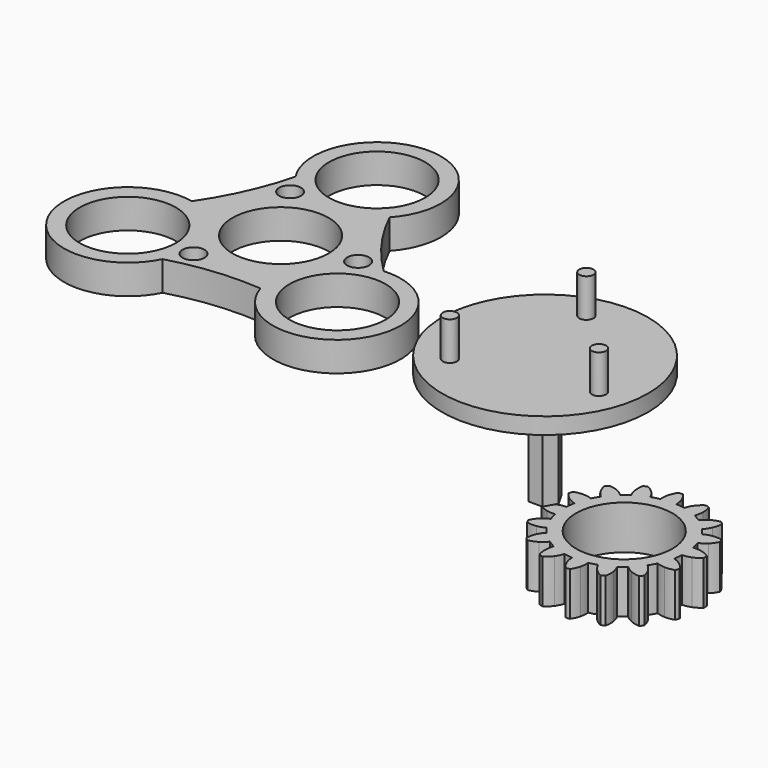
from build123d import *

# Parameters (mm, degrees)
F3_R     = 11.15
F4_DEPTH = 10.16
F0_R     = 11.15
F0_R_2   = 2.54
F5_DEPTH = 6.858
F1_R     = 23.8758575394
F1_R_2   = 1.651
F6_DEPTH = 3.81
F7_DEPTH = 12.7
F8_DEPTH = 25.4


# Not quite as in the source:
# - a feature names something its author has since deleted; it is built from what else it names


with BuildPart() as f4:
    # F3 (on offset) → F4 (new body)
    with BuildSketch(Plane.XY.offset(-25.4)):
        with BuildLine():
            ThreePointArc((46.6580232987, 12.782273917), (46.897414188, 11.8167860558), (47.2996218498, 10.9070037716))
            ThreePointArc((47.2996218498, 10.9070037716), (46.4885653807, 10.3281901983), (45.7204118752, 9.6935423112))
            ThreePointArc((45.7204118752, 9.6935423112), (44.9442772532, 10.316358652), (44.0729983828, 10.7971478738))
            ThreePointArc((44.0729983828, 10.7971478738), (43.042378943, 11.1427773384), (41.9651281062, 11.2882654524))
            ThreePointArc((41.9651281062, 11.2882654524), (41.6093843586, 10.9481924321), (41.3186545869, 10.5511036851))
            ThreePointArc((41.3186545869, 10.5511036851), (41.6034820024, 9.500074798), (42.0813519912, 8.5215919664))
            ThreePointArc((42.0813519912, 8.5215919664), (42.6719965427, 7.7212084197), (43.3917465765, 7.0345973968))
            ThreePointArc((43.3917465765, 7.0345973968), (42.86393047, 6.1894655098), (42.3971184001, 5.3091676965))
            ThreePointArc((42.3971184001, 5.3091676965), (41.4417220134, 5.5875611052), (40.4527752283, 5.698328438))
            ThreePointArc((40.4527752283, 5.698328438), (39.3683403522, 5.6232474415), (38.3174144619, 5.3454148845))
            ThreePointArc((38.3174144619, 5.3454148845), (38.1188904054, 4.8950911431), (38.0022504044, 4.4169715103))
            ThreePointArc((38.0022504044, 4.4169715103), (38.6676079659, 3.5549461664), (39.4835514363, 2.8338188328))
            ThreePointArc((39.4835514363, 2.8338188328), (40.3355293712, 2.3203907402), (41.263246359, 1.9614812827))
            ThreePointArc((41.263246359, 1.9614812827), (41.0990258325, 0.9786947508), (41.0046231044, -0.0132356266))
            ThreePointArc((41.0046231044, -0.0132356266), (40.015415392, -0.1216480228), (39.0593588755, -0.3977659014))
            ThreePointArc((39.0593588755, -0.3977659014), (38.0862039425, -0.8821269579), (37.2215969388, -1.5409826976))
            ThreePointArc((37.2215969388, -1.5409826976), (37.2105160613, -2.0329994527), (37.2857232139, -2.5193605914))
            ThreePointArc((37.2857232139, -2.5193605914), (38.2303162641, -3.0611468478), (39.2601132193, -3.4151335838))
            ThreePointArc((39.2601132193, -3.4151335838), (40.2437186203, -3.5634414495), (41.2381660604, -3.5400086302))
            ThreePointArc((41.2381660604, -3.5400086302), (41.4625422004, -4.5108294666), (41.7549207736, -5.46338))
            ThreePointArc((41.7549207736, -5.46338), (40.8824996427, -5.9420933966), (40.1048843326, -6.5630600425))
            ThreePointArc((40.1048843326, -6.5630600425), (39.3911633596, -7.3829615788), (38.8445038212, -8.3225356875))
            ThreePointArc((38.8445038212, -8.3225356875), (39.0225530859, -8.7813403654), (39.2781577848, -9.2018989356))
            ThreePointArc((39.2781577848, -9.2018989356), (40.3581805947, -9.3409640582), (41.4450537833, -9.2739189249))
            ThreePointArc((41.4450537833, -9.2739189249), (42.4105416445, -9.0345280356), (43.3203239288, -8.6323203737))
            ThreePointArc((43.3203239288, -8.6323203737), (43.8991375021, -9.4433768428), (44.5337853892, -10.2115303484))
            ThreePointArc((44.5337853892, -10.2115303484), (43.9109690483, -10.9876649703), (43.4301798266, -11.8589438407))
            ThreePointArc((43.4301798266, -11.8589438407), (43.0845503619, -12.8895632805), (42.939062248, -13.9668141173))
            ThreePointArc((42.939062248, -13.9668141173), (43.2791352683, -14.3225578649), (43.6762240152, -14.6132876366))
            ThreePointArc((43.6762240152, -14.6132876366), (44.7272529023, -14.3284602212), (45.705735734, -13.8505902324))
            ThreePointArc((45.705735734, -13.8505902324), (46.5061192806, -13.2599456808), (47.1927303036, -12.540195647))
            ThreePointArc((47.1927303036, -12.540195647), (48.0378621905, -13.0680117536), (48.9181600038, -13.5348238234))
            ThreePointArc((48.9181600038, -13.5348238234), (48.6397665951, -14.4902202101), (48.5289992624, -15.4791669952))
            ThreePointArc((48.5289992624, -15.4791669952), (48.6040802588, -16.5636018713), (48.8819128158, -17.6145277616))
            ThreePointArc((48.8819128158, -17.6145277616), (49.3322365572, -17.8130518182), (49.8103561901, -17.9296918191))
            ThreePointArc((49.8103561901, -17.9296918191), (50.672381534, -17.2643342577), (51.3935088675, -16.4483907873))
            ThreePointArc((51.3935088675, -16.4483907873), (51.9069369602, -15.5964128523), (52.2658464176, -14.6686958646))
            ThreePointArc((52.2658464176, -14.6686958646), (53.2486329496, -14.8329163911), (54.240563327, -14.9273191192))
            ThreePointArc((54.240563327, -14.9273191192), (54.3489757232, -15.9165268315), (54.6250936018, -16.8725833481))
            ThreePointArc((54.6250936018, -16.8725833481), (55.1094546582, -17.8457382811), (55.768310398, -18.7103452847))
            ThreePointArc((55.768310398, -18.7103452847), (56.260327153, -18.7214261623), (56.7466882918, -18.6462190096))
            ThreePointArc((56.7466882918, -18.6462190096), (57.2884745482, -17.7016259594), (57.6424612841, -16.6718290043))
            ThreePointArc((57.6424612841, -16.6718290043), (57.7907691499, -15.6882236032), (57.7673363305, -14.6937761632))
            ThreePointArc((57.7673363305, -14.6937761632), (58.7381571669, -14.4694000231), (59.6907077003, -14.17702145))
            ThreePointArc((59.6907077003, -14.17702145), (60.1694210969, -15.0494425809), (60.7903877428, -15.827057891))
            ThreePointArc((60.7903877428, -15.827057891), (61.6102892792, -16.5407788639), (62.5498633878, -17.0874384023))
            ThreePointArc((62.5498633878, -17.0874384023), (63.0086680657, -16.9093891377), (63.4292266359, -16.6537844387))
            ThreePointArc((63.4292266359, -16.6537844387), (63.5682917586, -15.5737616289), (63.5012466252, -14.4868884402))
            ThreePointArc((63.5012466252, -14.4868884402), (63.2618557359, -13.521400579), (62.8596480741, -12.6116182948))
            ThreePointArc((62.8596480741, -12.6116182948), (63.6707045432, -12.0328047215), (64.4388580487, -11.3981568344))
            ThreePointArc((64.4388580487, -11.3981568344), (65.2149926707, -12.0209731752), (66.0862715411, -12.501762397))
            ThreePointArc((66.0862715411, -12.501762397), (67.1168909809, -12.8473918616), (68.1941418176, -12.9928799756))
            ThreePointArc((68.1941418176, -12.9928799756), (68.5498855653, -12.6528069553), (68.8406153369, -12.2557182083))
            ThreePointArc((68.8406153369, -12.2557182083), (68.5557879215, -11.2046893212), (68.0779179327, -10.2262064896))
            ThreePointArc((68.0779179327, -10.2262064896), (67.4872733812, -9.4258229429), (66.7675233473, -8.73921192))
            ThreePointArc((66.7675233473, -8.73921192), (67.2953394539, -7.894080033), (67.7621515238, -7.0137822197))
            ThreePointArc((67.7621515238, -7.0137822197), (68.7175479105, -7.2921756284), (69.7064946956, -7.4029429612))
            ThreePointArc((69.7064946956, -7.4029429612), (70.7909295717, -7.3278619647), (71.841855462, -7.0500294077))
            ThreePointArc((71.841855462, -7.0500294077), (72.0403795185, -6.5997056663), (72.1570195195, -6.1215860335))
            ThreePointArc((72.1570195195, -6.1215860335), (71.491661958, -5.2595606896), (70.6757184876, -4.538433356))
            ThreePointArc((70.6757184876, -4.538433356), (69.8237405526, -4.0250052634), (68.8960235649, -3.6660958059))
            ThreePointArc((68.8960235649, -3.6660958059), (69.0602440914, -2.683309274), (69.1546468195, -1.6913788966))
            ThreePointArc((69.1546468195, -1.6913788966), (70.1438545319, -1.5829665003), (71.0999110484, -1.3068486218))
            ThreePointArc((71.0999110484, -1.3068486218), (72.0730659814, -0.8224875653), (72.9376729851, -0.1636318256))
            ThreePointArc((72.9376729851, -0.1636318256), (72.9487538626, 0.3283849295), (72.87354671, 0.8147460683))
            ThreePointArc((72.87354671, 0.8147460683), (71.9289536598, 1.3565323246), (70.8991567046, 1.7105190606))
            ThreePointArc((70.8991567046, 1.7105190606), (69.9155513036, 1.8588269263), (68.9211038635, 1.835394107))
            ThreePointArc((68.9211038635, 1.835394107), (68.6967277235, 2.8062149434), (68.4043491503, 3.7587654768))
            ThreePointArc((68.4043491503, 3.7587654768), (69.2767702812, 4.2374788734), (70.0543855913, 4.8584455193))
            ThreePointArc((70.0543855913, 4.8584455193), (70.7681065642, 5.6783470556), (71.3147661027, 6.6179211643))
            ThreePointArc((71.3147661027, 6.6179211643), (71.136716838, 7.0767258422), (70.8811121391, 7.4972844124))
            ThreePointArc((70.8811121391, 7.4972844124), (69.8010893292, 7.636349535), (68.7142161406, 7.5693044017))
            ThreePointArc((68.7142161406, 7.5693044017), (67.7487282794, 7.3299135124), (66.8389459951, 6.9277058505))
            ThreePointArc((66.8389459951, 6.9277058505), (66.2601324218, 7.7387623196), (65.6254845347, 8.5069158252))
            ThreePointArc((65.6254845347, 8.5069158252), (66.2483008756, 9.2830504471), (66.7290900973, 10.1543293175))
            ThreePointArc((66.7290900973, 10.1543293175), (67.074719562, 11.1849487573), (67.2202076759, 12.2621995941))
            ThreePointArc((67.2202076759, 12.2621995941), (66.8801346556, 12.6179433417), (66.4830459087, 12.9086731134))
            ThreePointArc((66.4830459087, 12.9086731134), (65.4320170216, 12.623845698), (64.4535341899, 12.1459757092))
            ThreePointArc((64.4535341899, 12.1459757092), (63.6531506432, 11.5553311576), (62.9665396203, 10.8355811238))
            ThreePointArc((62.9665396203, 10.8355811238), (62.1214077334, 11.3633972304), (61.2411099201, 11.8302093002))
            ThreePointArc((61.2411099201, 11.8302093002), (61.5195033288, 12.7856056869), (61.6302706615, 13.774552472))
            ThreePointArc((61.6302706615, 13.774552472), (61.5551896651, 14.8589873482), (61.277357108, 15.9099132384))
            ThreePointArc((61.277357108, 15.9099132384), (60.8270333666, 16.108437295), (60.3489137338, 16.2250772959))
            ThreePointArc((60.3489137338, 16.2250772959), (59.4868883899, 15.5597197345), (58.7657610564, 14.7437762641))
            ThreePointArc((58.7657610564, 14.7437762641), (58.2523329637, 13.8917983291), (57.8934235063, 12.9640813414))
            ThreePointArc((57.8934235063, 12.9640813414), (56.9106369743, 13.1283018679), (55.9187065969, 13.222704596))
            ThreePointArc((55.9187065969, 13.222704596), (55.8102942007, 14.2119123083), (55.5341763221, 15.1679688249))
            ThreePointArc((55.5341763221, 15.1679688249), (55.0498152657, 16.1411237579), (54.3909595259, 17.0057307615))
            ThreePointArc((54.3909595259, 17.0057307615), (53.8989427709, 17.0168116391), (53.4125816321, 16.9416044864))
            ThreePointArc((53.4125816321, 16.9416044864), (52.8707953757, 15.9970114362), (52.5168086398, 14.9672144811))
            ThreePointArc((52.5168086398, 14.9672144811), (52.368500774, 13.98360908), (52.3919335934, 12.98916164))
            ThreePointArc((52.3919335934, 12.98916164), (51.421112757, 12.7647854999), (50.4685622236, 12.4724069268))
            ThreePointArc((50.4685622236, 12.4724069268), (49.989848827, 13.3448280577), (49.3688821811, 14.1224433678))
            ThreePointArc((49.3688821811, 14.1224433678), (48.5489806447, 14.8361643407), (47.6094065361, 15.3828238791))
            ThreePointArc((47.6094065361, 15.3828238791), (47.1506018582, 15.2047746145), (46.730043288, 14.9491699155))
            ThreePointArc((46.730043288, 14.9491699155), (46.5909781653, 13.8691471057), (46.6580232987, 12.782273917))
        make_face()
        with Locations((55.0796349619, -0.8523072616)):
            Circle(F3_R, mode=Mode.SUBTRACT)
    extrude(amount=-F4_DEPTH)


with BuildPart() as f5:
    # F0 (on Top) → F5 (new body)
    with BuildSketch(Plane.XY):
        with BuildLine():
            ThreePointArc((-39.3561690708, 21.9977449829), (-42.8395859433, 11.9927540801), (-48.0209129825, 2.7521974852))
            ThreePointArc((-48.0209129825, 2.7521974852), (-64.5879284102, -18.0924816154), (-37.9620499011, -18.2634804685))
            ThreePointArc((-37.9620499011, -18.2634804685), (-27.5557651784, -16.2777125207), (-16.9625449025, -16.1445950645))
            ThreePointArc((-16.9625449025, -16.1445950645), (9.3729844462, -20.0697117395), (-3.7918654575, 3.074474874))
            ThreePointArc((-3.7918654575, 3.074474874), (-10.7147333077, 11.0936978289), (-16.1266265444, 20.2011369677))
            ThreePointArc((-16.1266265444, 20.2011369677), (-25.8951404654, 44.9709327433), (-39.3561690708, 21.9977449829))
        make_face()
        with Locations((-51.160162566, -11.8265864704)):
            Circle(F0_R, mode=Mode.SUBTRACT)
        with Locations((-34.8965979527, -13.110404163)):
            Circle(F0_R_2, mode=Mode.SUBTRACT)
        with Locations((-27.0366948098, 2.2695797961)):
            Circle(F0_R, mode=Mode.SUBTRACT)
        with Locations((-2.7673228489, -11.5738729749)):
            Circle(F0_R, mode=Mode.SUBTRACT)
        with Locations((-9.7872864199, 3.1526959827)):
            Circle(F0_R_2, mode=Mode.SUBTRACT)
        with Locations((-36.4262000568, 16.7664475687)):
            Circle(F0_R_2, mode=Mode.SUBTRACT)
        with Locations((-27.036805868, 30.2095797961)):
            Circle(F0_R, mode=Mode.SUBTRACT)
    extrude(amount=F5_DEPTH)


with BuildPart() as f6:
    # F1 (on Top) → F6 (new body)
    with BuildSketch(Plane.XY):
        with Locations((35.9901546764, 0.0754770181)):
            Circle(F1_R)
        with Locations((23.3627118705, -11.7088206777)):
            Circle(F1_R_2, mode=Mode.SUBTRACT)
        with Locations((52.5093772497, -4.9680603887)):
            Circle(F1_R_2, mode=Mode.SUBTRACT)
        with Locations((32.0983749091, 16.9033121208)):
            Circle(F1_R_2, mode=Mode.SUBTRACT)
        Polygon((39.1651546764, 0.0754770181), (37.5776546764, -2.6741536389), (34.4026546764, -2.6741536389), (32.8151546764, 0.0754770181), (34.4026546764, 2.8251076752), (37.5776546764, 2.8251076752), align=None, mode=Mode.SUBTRACT)
        Polygon((34.4026546764, -2.6741536389), (37.5776546764, -2.6741536389), (39.1651546764, 0.0754770181), (37.5776546764, 2.8251076752), (34.4026546764, 2.8251076752), (32.8151546764, 0.0754770181), align=None)
    extrude(amount=F6_DEPTH)

    # F1 (on Top) → F7 (join)
    with BuildSketch(Plane.XY):
        with Locations((32.0983749091, 16.9033121208)):
            Circle(F1_R_2)
        with Locations((23.3627118705, -11.7088206777)):
            Circle(F1_R_2)
        with Locations((52.5093772497, -4.9680603887)):
            Circle(F1_R_2)
    extrude(amount=F7_DEPTH)

    # F1 (on Top) → F8 (join)
    with BuildSketch(Plane.XY):
        Polygon((34.4026546764, -2.6741536389), (37.5776546764, -2.6741536389), (39.1651546764, 0.0754770181), (37.5776546764, 2.8251076752), (34.4026546764, 2.8251076752), (32.8151546764, 0.0754770181), align=None)
    extrude(amount=-F8_DEPTH)


solid = Compound([f4.part, f5.part, f6.part])
